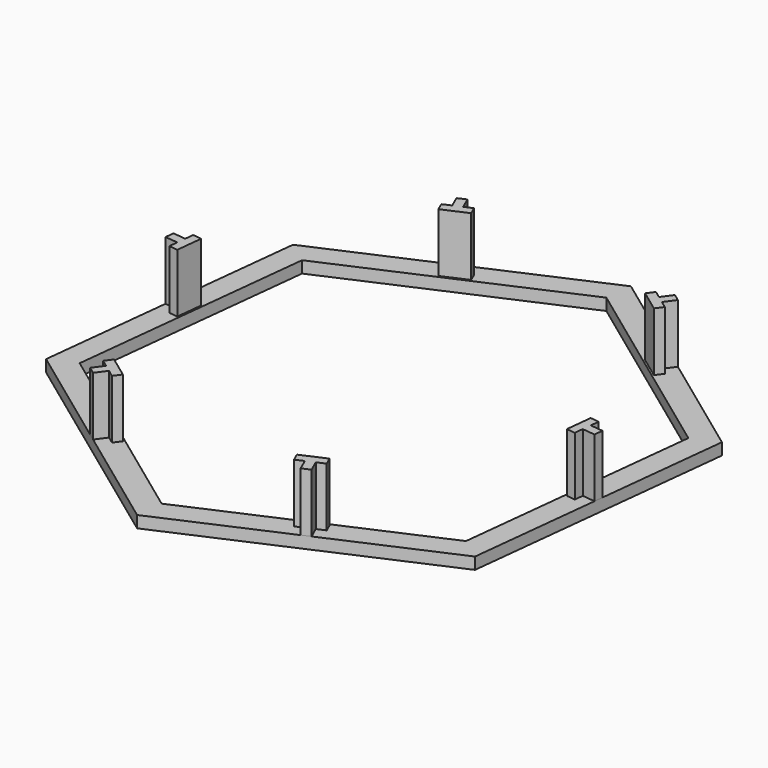
from build123d import *

# Parameters (mm, degrees)
F1_DEPTH = 2
F3_DEPTH = 10


# Not quite as in the source:
# - a feature names something its author has since deleted; it is built from what else it names


with BuildPart() as f1:
    # F0 (on Top) → F1 (new body)
    with BuildSketch(Plane.XY):
        Polygon((-5.0628672683, -46.2001158912), (37.4790403854, -27.4846296159), (42.5419076537, 18.7154862752), (5.0628672683, 46.2001158912), (-37.4790403854, 27.4846296159), (-42.5419076537, -18.7154862752), align=None)
        Polygon((-38.3141404334, -16.8555621733), (-33.7544152539, 24.7532378529), (4.5597251795, 41.6088000262), (38.3141404334, 16.8555621733), (33.7544152539, -24.7532378529), (-4.5597251795, -41.6088000262), align=None, mode=Mode.SUBTRACT)
    extrude(amount=F1_DEPTH)

    # F2 (on face) → F3 (join)
    with BuildSketch(Plane.XY.offset(2)):
        Polygon((-15.5215827184, 37.1443867888), (-16.8945903987, 36.5403587183), (-16.0086825619, 34.5266141206), (-17.3816902422, 33.9225860501), (-16.7776621717, 32.5495783698), (-12.6586391309, 34.3616625813), (-13.2626672014, 35.7346702616), (-14.6356748817, 35.1306421911), align=None)
        Polygon((24.4071912079, 32.0142783355), (23.1975837141, 32.9013238309), (21.8965836541, 31.12723284), (20.6869761604, 32.0142783355), (19.7999306649, 30.8046708417), (23.4287531463, 28.1435343554), (24.3157986417, 29.3531418491), (23.1061911479, 30.2401873446), align=None)
        Polygon((37.7418660296, -4.8904548465), (39.9287739263, -5.1301084533), (40.0921741128, -3.6390348874), (37.905266216, -3.3993812806), (38.0686664025, -1.9083077146), (36.5775928366, -1.7449075281), (36.0873922772, -6.218128226), (37.5784658431, -6.3815284124), align=None)
        Polygon((14.6356748817, -35.1306421911), (15.5215827184, -37.1443867888), (16.8945903987, -36.5403587183), (16.0086825619, -34.5266141206), (17.3816902422, -33.9225860501), (16.7776621717, -32.5495783698), (12.6586391309, -34.3616625813), (13.2626672014, -35.7346702616), align=None)
        Polygon((-23.1061911479, -30.2401873446), (-24.4071912079, -32.0142783355), (-23.1975837141, -32.9013238309), (-21.8965836541, -31.12723284), (-20.6869761604, -32.0142783355), (-19.7999306649, -30.8046708417), (-23.4287531463, -28.1435343554), (-24.3157986417, -29.3531418491), align=None)
        Polygon((-39.9287739263, 5.1301084533), (-40.0921741128, 3.6390348874), (-37.905266216, 3.3993812806), (-38.0686664025, 1.9083077146), (-36.5775928366, 1.7449075281), (-36.0873922772, 6.218128226), (-37.5784658431, 6.3815284124), (-37.7418660296, 4.8904548465), align=None)
    extrude(amount=F3_DEPTH)


solid = f1.part
